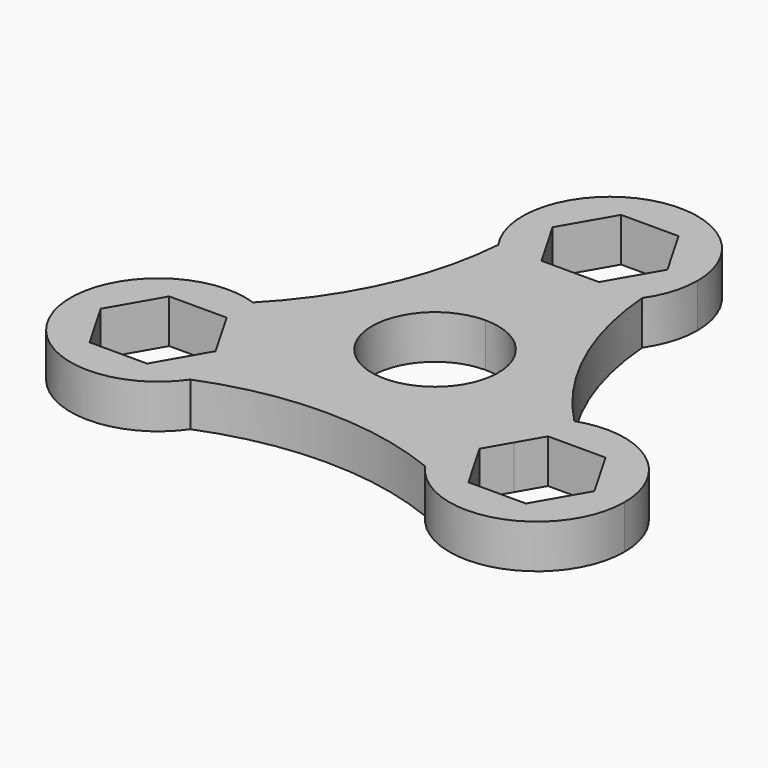
from build123d import *

# Parameters (mm, degrees)
F1_DEPTH = 7.62


# Not quite as in the source:
# - a feature names something its author has since deleted; it is built from what else it names


with BuildPart() as f1:
    # F0 (on Top) → F1 (new body)
    with BuildSketch(Plane.XY):
        with BuildLine():
            ThreePointArc((-12.5356913124, 29.4331641691), (-7.0772530666, 24.60295999), (0, 22.86))
            ThreePointArc((0, 22.86), (7.0772530666, 24.60295999), (12.5356913124, 29.4331641691))
            ThreePointArc((12.5356913124, 29.4331641691), (14.5482221526, 33.5605251185), (15.24, 38.1))
            ThreePointArc((15.24, 38.1), (-4.5394748815, 52.6482221526), (-12.5356913124, 29.4331641691))
        make_face()
        Polygon((5.0038, 29.4331641691), (0, 29.4331641691), (-5.0038, 29.4331641691), (-10.0076, 38.1), (-5.0038, 46.7668358309), (5.0038, 46.7668358309), (10.0076, 38.1), align=None, mode=Mode.SUBTRACT)
        with BuildLine():
            ThreePointArc((27.9917678842, -4.654876327), (23.2845420207, -7.3046359495), (19.7973407305, -11.43))
            ThreePointArc((19.7973407305, -11.43), (17.7681618263, -19.6694390603), (20.4598765718, -27.7168358309))
            ThreePointArc((20.4598765718, -27.7168358309), (37.5350427657, -33.5982221526), (48.2355678842, -19.05))
            ThreePointArc((48.2355678842, -19.05), (41.8273199187, -6.6299454107), (27.9917678842, -4.654876327))
        make_face()
        Polygon((22.9879678842, -19.05), (25.4898678842, -14.7165820845), (27.9917678842, -10.3831641691), (37.9993678842, -10.3831641691), (43.0031678842, -19.05), (37.9993678842, -27.7168358309), (27.9917678842, -27.7168358309), align=None, mode=Mode.SUBTRACT)
        with BuildLine():
            ThreePointArc((-17.7555678842, -19.05), (-18.2748582915, -15.1055977526), (-19.7973407305, -11.43))
            ThreePointArc((-19.7973407305, -11.43), (-23.2845420207, -7.3046359495), (-27.9917678842, -4.654876327))
            ThreePointArc((-27.9917678842, -4.654876327), (-47.4825252222, -23.7813493938), (-20.4598765718, -27.7168358309))
            ThreePointArc((-20.4598765718, -27.7168358309), (-18.4473457316, -23.5894748815), (-17.7555678842, -19.05))
        make_face()
        Polygon((-27.9917678842, -10.3831641691), (-25.4898678842, -14.7165820845), (-22.9879678842, -19.05), (-27.9917678842, -27.7168358309), (-37.9993678842, -27.7168358309), (-43.0031678842, -19.05), (-37.9993678842, -10.3831641691), align=None, mode=Mode.SUBTRACT)
        with BuildLine():
            ThreePointArc((-9.5247205959, -5.4991), (-9.5247205959, 5.4991), (0, 10.9982))
            Line((0, 10.9982), (0, 22.86))
            ThreePointArc((0, 22.86), (-7.0772530666, 24.60295999), (-12.5356913124, 29.4331641691))
            ThreePointArc((-12.5356913124, 29.4331641691), (-17.2521616486, 11.0236496258), (-27.9917678842, -4.654876327))
            ThreePointArc((-27.9917678842, -4.654876327), (-23.2845420207, -7.3046359495), (-19.7973407305, -11.43))
            Line((-19.7973407305, -11.43), (-9.5247205959, -5.4991))
        make_face()
        with BuildLine():
            Line((0, 22.86), (0, 10.9982))
            ThreePointArc((0, 10.9982), (7.7769018008, 7.7769018008), (10.9982, 0))
            ThreePointArc((10.9982, 0), (10.6234454227, -2.8465436218), (9.5247205959, -5.4991))
            Line((9.5247205959, -5.4991), (19.7973407305, -11.43))
            ThreePointArc((19.7973407305, -11.43), (23.2845420207, -7.3046359495), (27.9917678842, -4.654876327))
            ThreePointArc((27.9917678842, -4.654876327), (17.2521616486, 11.0236496258), (12.5356913124, 29.4331641691))
            ThreePointArc((12.5356913124, 29.4331641691), (7.0772530666, 24.60295999), (0, 22.86))
        make_face()
        with BuildLine():
            ThreePointArc((9.5247205959, -5.4991), (0, -10.9982), (-9.5247205959, -5.4991))
            Line((-9.5247205959, -5.4991), (-19.7973407305, -11.43))
            ThreePointArc((-19.7973407305, -11.43), (-18.2748582915, -15.1055977526), (-17.7555678842, -19.05))
            ThreePointArc((-17.7555678842, -19.05), (-18.4473457316, -23.5894748815), (-20.4598765718, -27.7168358309))
            ThreePointArc((-20.4598765718, -27.7168358309), (0, -23.7392913379), (20.4598765718, -27.7168358309))
            ThreePointArc((20.4598765718, -27.7168358309), (17.7681618263, -19.6694390603), (19.7973407305, -11.43))
            Line((19.7973407305, -11.43), (9.5247205959, -5.4991))
        make_face()
    extrude(amount=F1_DEPTH)


solid = f1.part
